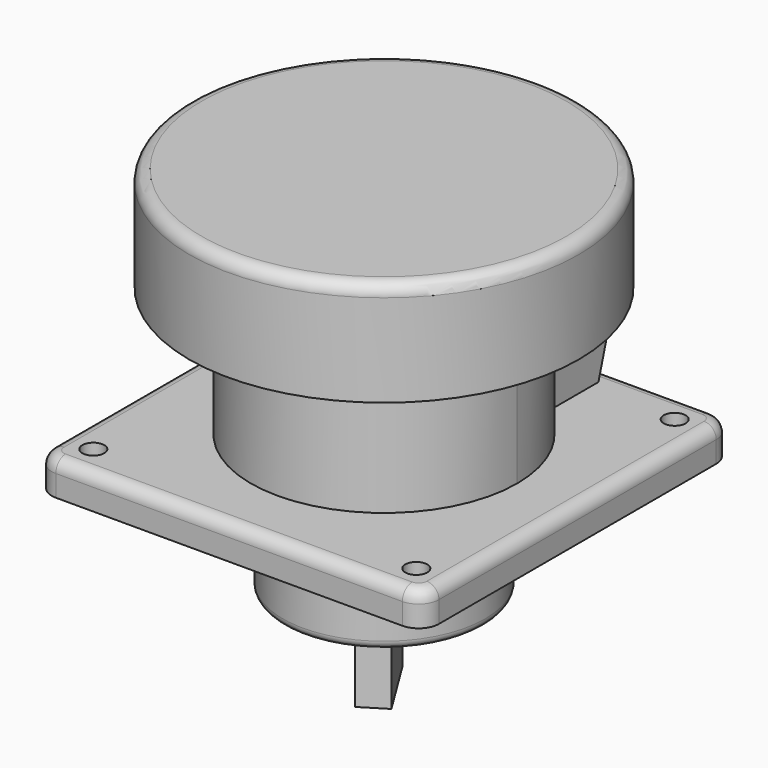
from build123d import *

# Parameters (mm, degrees)
F0_R         = 2.7
F1_DEPTH     = 8.25
F0_W         = 37.2
F0_H         = 3
F2_DEPTH     = 40
F3_R         = 47.9
F4_DEPTH     = 25.7
F5_R         = 3
F5_2_R       = 3
F6_T1_DEPTH  = 20.75
F6_T3_DEPTH  = 62.2
F6_T6_ANGLE  = 90
F6_T8_ANGLE  = 90
F6_T10_ANGLE = 90
F6_T12_ANGLE = 90
F8_DEPTH     = 66.501
F9_R         = 28.6
F9_R_2       = 24.9
F10_DEPTH    = 7.3
F11_DEPTH    = 25.6
F12_R        = 2
F14_DEPTH    = 16


# Not quite as in the source:
# - a fillet or chamfer that OpenCascade refuses, or shapes differently, is made with other operations: its cross-section is extruded or revolved along the edge and cut away or added


with BuildPart() as f1:
    # F0 (on Top) → F1 (new body)
    with BuildSketch(Plane.XY):
        with BuildLine():
            Line((-47.6, -47.6), (47.6, -47.6))
            Line((47.6, -47.6), (47.6, 47.6))
            Line((47.6, 47.6), (18.6, 47.6))
            Line((18.6, 47.6), (18.6, 29.6))
            Line((18.6, 29.6), (18.6, 26.955565))
            ThreePointArc((18.6, 26.955565), (28.997521, 15.2219), (32.75, 0))
            ThreePointArc((32.75, 0), (-15.2219, -28.997521), (-18.6, 26.955565))
            Line((-18.6, 26.955565), (-18.6, 29.6))
            Line((-18.6, 29.6), (-18.6, 47.6))
            Line((-18.6, 47.6), (-47.6, 47.6))
            Line((-47.6, 47.6), (-47.6, -47.6))
        make_face()
        with Locations((-39.7, -39.7)):
            Circle(F0_R, mode=Mode.SUBTRACT)
        with Locations((39.7, -39.7)):
            Circle(F0_R, mode=Mode.SUBTRACT)
        with Locations((-39.7, 39.7)):
            Circle(F0_R, mode=Mode.SUBTRACT)
        with Locations((39.7, 39.7)):
            Circle(F0_R, mode=Mode.SUBTRACT)
    extrude(amount=F1_DEPTH)

    # F0 (on Top) → F2 (join)
    with BuildSketch(Plane.XY):
        with Locations((0, 49.1)):
            Rectangle(F0_W, F0_H)
        with BuildLine():
            Line((18.6, 29.6), (18.6, 47.6))
            Line((18.6, 47.6), (-18.6, 47.6))
            Line((-18.6, 47.6), (-18.6, 29.6))
            Line((-18.6, 29.6), (-18.6, 26.955565))
            ThreePointArc((-18.6, 26.955565), (0, 32.75), (18.6, 26.955565))
            Line((18.6, 26.955565), (18.6, 29.6))
        make_face()
        with BuildLine():
            ThreePointArc((32.75, 0), (28.997521, 15.2219), (18.6, 26.955565))
            ThreePointArc((18.6, 26.955565), (0, 32.75), (-18.6, 26.955565))
            ThreePointArc((-18.6, 26.955565), (-15.2219, -28.997521), (32.75, 0))
        make_face()
    extrude(amount=F2_DEPTH)

    # F5#2
    f5_2_edges = [f1.edges().sort_by_distance(p)[0] for p in [
        (-47.6, 0, 8.25),
        (-33.1, 47.6, 8.25),
        (0, -47.6, 8.25),
        (47.6, 0, 8.25),
        (33.1, 47.6, 8.25),
    ]]
    fillet(f5_2_edges, radius=F5_2_R)

    # F6: fillet of radius 5 on 5 edges, made by hand

    # F6_s2 → F6_t1 (cut)
    with BuildSketch(Plane.XY.offset(-12.5)):
        with BuildLine():
            ThreePointArc((-42.6, -47.6), (-46.135534, -46.135534), (-47.6, -42.6))
            Line((-47.6, -42.6), (-47.6, -47.6))
            Line((-47.6, -47.6), (-42.6, -47.6))
        make_face()
        with BuildLine():
            ThreePointArc((42.6, -47.6), (46.135534, -46.135534), (47.6, -42.6))
            Line((47.6, -42.6), (47.6, -47.6))
            Line((47.6, -47.6), (42.6, -47.6))
        make_face()
        with BuildLine():
            ThreePointArc((47.6, 42.6), (46.135534, 46.135534), (42.6, 47.6))
            Line((42.6, 47.6), (47.6, 47.6))
            Line((47.6, 47.6), (47.6, 42.6))
        make_face()
        with BuildLine():
            ThreePointArc((-47.6, 42.6), (-46.135534, 46.135534), (-42.6, 47.6))
            Line((-42.6, 47.6), (-47.6, 47.6))
            Line((-47.6, 47.6), (-47.6, 42.6))
        make_face()
    extrude(amount=F6_T1_DEPTH, mode=Mode.SUBTRACT)

    # F6_s4 → F6_t3 (cut)
    with BuildSketch(Plane.YZ.offset(-31.1)):
        with BuildLine():
            ThreePointArc((50.6, 35), (49.135534, 38.535534), (45.6, 40))
            Line((45.6, 40), (50.6, 40))
            Line((50.6, 40), (50.6, 35))
        make_face()
    extrude(amount=F6_T3_DEPTH, mode=Mode.SUBTRACT)

    # F6_s5 → F6_t6 (revolve, cut)
    with BuildSketch(Plane.YZ.offset(-42.6)):
        with BuildLine():
            ThreePointArc((44.6, 8.25), (46.72132, 7.37132), (47.6, 5.25))
            Line((47.6, 5.25), (47.6, 8.25))
            Line((47.6, 8.25), (44.6, 8.25))
        make_face()
    revolve(axis=Axis((-42.6, 42.6, 8.25), (0, 0, 1)), revolution_arc=F6_T6_ANGLE, mode=Mode.SUBTRACT)

    # F6_s7 → F6_t8 (revolve, cut)
    with BuildSketch(Plane.XZ.offset(-42.6)):
        with BuildLine():
            ThreePointArc((44.6, 8.25), (46.72132, 7.37132), (47.6, 5.25))
            Line((47.6, 5.25), (47.6, 8.25))
            Line((47.6, 8.25), (44.6, 8.25))
        make_face()
    revolve(axis=Axis((42.6, 42.6, 8.25), (0, 0, 1)), revolution_arc=F6_T8_ANGLE, mode=Mode.SUBTRACT)

    # F6_s9 → F6_t10 (revolve, cut)
    with BuildSketch(Plane.YZ.offset(42.6)):
        with BuildLine():
            ThreePointArc((-44.6, 8.25), (-46.72132, 7.37132), (-47.6, 5.25))
            Line((-47.6, 5.25), (-47.6, 8.25))
            Line((-47.6, 8.25), (-44.6, 8.25))
        make_face()
    revolve(axis=Axis((42.6, -42.6, 8.25), (0, 0, 1)), revolution_arc=F6_T10_ANGLE, mode=Mode.SUBTRACT)

    # F6_s11 → F6_t12 (revolve, cut)
    with BuildSketch(Plane.XZ.offset(42.6)):
        with BuildLine():
            ThreePointArc((-44.6, 8.25), (-46.72132, 7.37132), (-47.6, 5.25))
            Line((-47.6, 5.25), (-47.6, 8.25))
            Line((-47.6, 8.25), (-44.6, 8.25))
        make_face()
    revolve(axis=Axis((-42.6, -42.6, 8.25), (0, 0, 1)), revolution_arc=F6_T12_ANGLE, mode=Mode.SUBTRACT)

    # F7 (on face) → F8 (cut, through all)
    with BuildSketch(Plane(origin=(-18.6, 0, 0), x_dir=(0, -1, 0), z_dir=(-1, 0, 0))):
        with BuildLine():
            Line((-42.644739, 8.25), (-50.6, 35))
            Line((-50.6, 35), (-50.6, 0))
            Line((-50.6, 0), (-47.6, 0))
            Line((-47.6, 0), (-47.6, 5.25))
            ThreePointArc((-47.6, 5.25), (-46.72132, 7.37132), (-44.6, 8.25))
            Line((-44.6, 8.25), (-42.644739, 8.25))
        make_face()
    extrude(amount=-F8_DEPTH, mode=Mode.SUBTRACT)

    # F9 (on face) → F10 (join)
    with BuildSketch(Plane.XY):
        Circle(F9_R)
        Circle(F9_R_2, mode=Mode.SUBTRACT)
    extrude(amount=-F10_DEPTH)

    # F9 (on face) → F11 (join)
    with BuildSketch(Plane.XY):
        Circle(F9_R_2)
    extrude(amount=-F11_DEPTH)

    # F12
    f12_edges = [f1.edges().sort_by_distance(p)[0] for p in [
        (-28.6, 0, -7.3),
        (-24.9, 0, -25.6),
    ]]
    fillet(f12_edges, radius=F12_R)

    # F13 (on face) → F14 (join)
    with BuildSketch(Plane(origin=(0, 0, -25.6), x_dir=(1, 0, 0), z_dir=(0, 0, -1))):
        Polygon((12.642668, 13.529758), (6.625608, 17.25864), (-2.778482, 2.083861), (3.238578, -1.645021), (12.270656, 12.929466), align=None)
    extrude(amount=F14_DEPTH)


with BuildPart() as f4:
    # F3 (on face) → F4 (new body)
    with BuildSketch(Plane.XY.offset(40)):
        Circle(F3_R)
    extrude(amount=F4_DEPTH)

    # F5
    f5_edges = [f4.edges().sort_by_distance(p)[0] for p in [
        (-47.9, 0, 65.7),
    ]]
    fillet(f5_edges, radius=F5_R)


solid = Compound([f1.part, f4.part])
